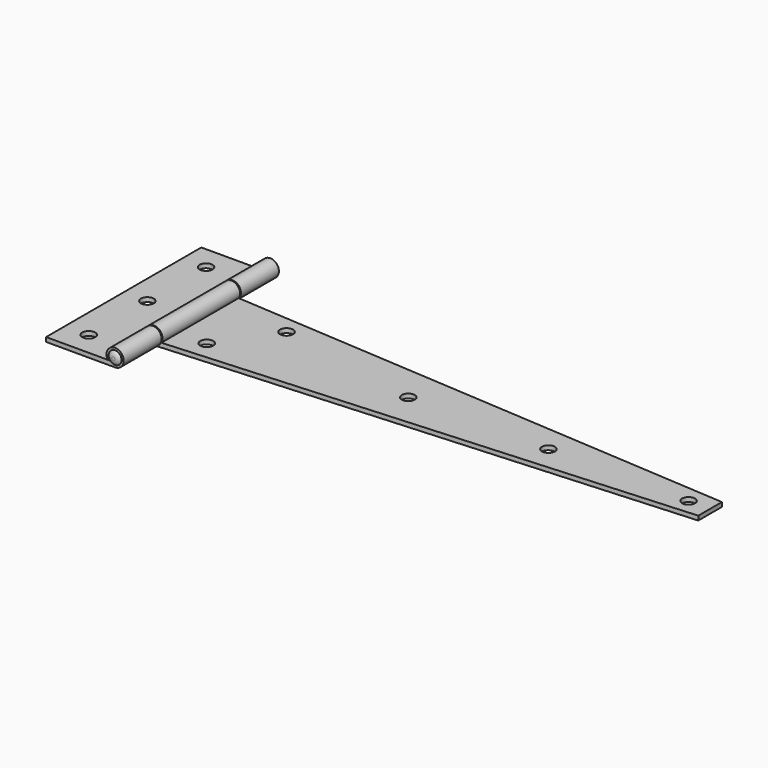
from build123d import *

# Parameters (mm, degrees)
F2_DEPTH  = 90
F3_W      = 67.9701848628
F3_H      = 46
F4_DEPTH  = 12.5
F6_D      = 6
F7_R      = 1.95
F8_DEPTH  = 90
F9_R      = 3
F10_DEPTH = 1
F12_R     = 3
F13_DEPTH = 1
F16_DEPTH = 2
F18_DEPTH = 45
F20_D     = 6


# Not quite as in the source:
# - a fillet or chamfer that OpenCascade refuses, or shapes differently, is made with other operations: its cross-section is extruded or revolved along the edge and cut away or added


with BuildPart() as f2:
    # F1 (on Front) → F2 (new body)
    with BuildSketch(Plane.XZ):
        with BuildLine():
            Line((0, 2), (0, 0))
            Line((0, 0), (32, 0))
            ThreePointArc((32, 0), (34.0493901532, 7.4351128075), (28.4800568186, 2.1))
            Line((28.4800568186, 2.1), (31.3755002002, 2.1))
            ThreePointArc((31.3755002002, 2.1), (32.316227766, 5.9748417658), (32, 2))
            Line((32, 2), (0, 2))
        make_face()
    extrude(amount=F2_DEPTH)

    # F3 (on face) → F4 (cut, symmetric)
    with BuildSketch(Plane.XY.offset(2)):
        with Locations((58.1850924314, -45)):
            Rectangle(F3_W, F3_H)
    extrude(amount=F4_DEPTH, both=True, mode=Mode.SUBTRACT)

    # F6 (through all)
    with Locations(Plane.XY.offset(2)):
        with Locations((11, -11), (11, -45), (11, -79)):
            Hole(F6_D / 2)


with BuildPart() as f8:
    # F7 (on Front) → F8 (new body)
    with BuildSketch(Plane.XZ):
        with Locations((32, 4)):
            Circle(F7_R)
    extrude(amount=F8_DEPTH)

    # F9 (on face) → F10 (join)
    with BuildSketch(Plane(origin=(0, 0, 0), x_dir=(-1, 0, 0), z_dir=(0, 1, 0))):
        with Locations((-32, 4)):
            Circle(F9_R)
    extrude(amount=F10_DEPTH)

    # F11: fillet of radius 3 on 1 edges, made by hand

    # F11_s1 → F11_t2 (revolve, cut)
    with BuildSketch(Plane.XY.offset(4)):
        with BuildLine():
            ThreePointArc((29, 0), (30.0113231061, 0.7386127875), (31.2360679775, 1))
            Line((31.2360679775, 1), (29, 1))
            Line((29, 1), (29, 0))
        make_face()
    revolve(axis=Axis((32, 1, 4), (0, 1, 0)), mode=Mode.SUBTRACT)

    # F12 (on face) → F13 (join)
    with BuildSketch(Plane.XZ.offset(90)):
        with Locations((32, 4)):
            Circle(F12_R)
    extrude(amount=F13_DEPTH)

    # F14: fillet of radius 3 on 1 edges, made by hand

    # F14_s1 → F14_t2 (revolve, cut)
    with BuildSketch(Plane.XY.offset(4)):
        with BuildLine():
            ThreePointArc((35, -90), (33.9886768939, -90.7386127875), (32.7639320225, -91))
            Line((32.7639320225, -91), (35, -91))
            Line((35, -91), (35, -90))
        make_face()
    revolve(axis=Axis((32, -91, 4), (0, -1, 0)), mode=Mode.SUBTRACT)


with BuildPart() as f16:
    # F15 (on Top) → F16 (new body)
    with BuildSketch(Plane.XY):
        Polygon((272, -38.15), (34, -22.5), (32, -22.5), (32, -67.5), (34, -67.5), (272, -51.85), align=None)
    extrude(amount=F16_DEPTH)

    # F17 (on face) → F18 (join)
    with BuildSketch(Plane(origin=(0, -22.5, 0), x_dir=(-1, 0, 0), z_dir=(0, 1, 0))):
        with BuildLine():
            Line((-32, 2), (-32, 0))
            ThreePointArc((-32, 0), (-29.9506098468, 7.4351128075), (-35.5199431814, 2.1))
            Line((-35.5199431814, 2.1), (-32.6244997998, 2.1))
            ThreePointArc((-32.6244997998, 2.1), (-31.683772234, 5.9748417658), (-32, 2))
        make_face()
    extrude(amount=-F18_DEPTH)

    # F20 (through all)
    with Locations(Plane.XY.offset(2)):
        with Locations((48.5199431814, -57.5), (65.5199431814, -32.5), (197, -45), (132, -45), (262, -45)):
            Hole(F20_D / 2)


solid = Compound([f2.part, f8.part, f16.part])
